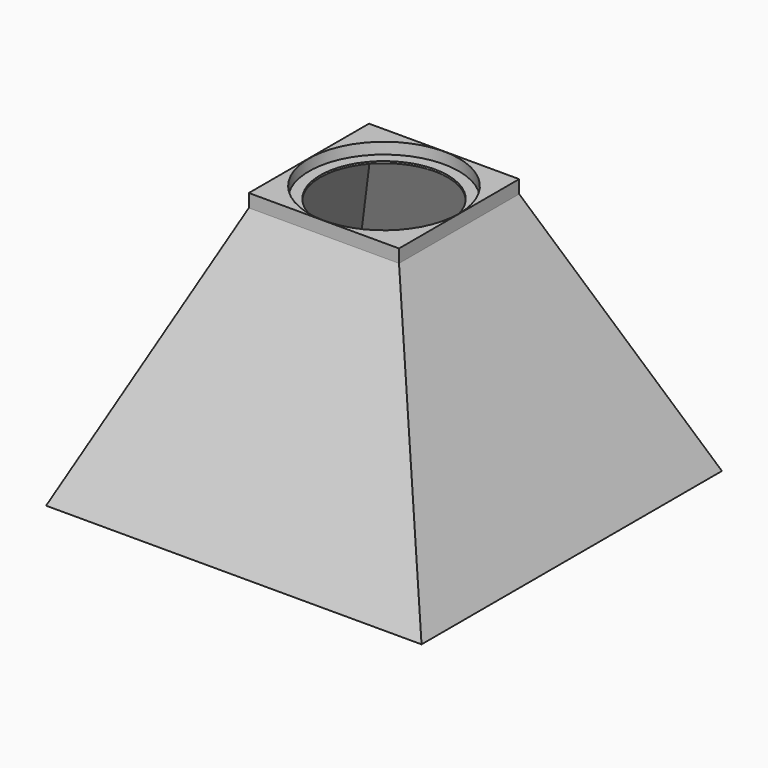
from build123d import *

# Parameters (mm, degrees)
F0_W      = 100
F0_H      = 100
F4_W      = 40
F4_H      = 40
F8_W      = 94
F8_H      = 94
F9_W      = 34
F9_H      = 34
F11_W     = 40
F11_H     = 40
F11_R     = 17
F12_DEPTH = 3.5
F13_R     = 19.95
F14_DEPTH = 3


with BuildPart() as f7:
    # F0 (on Top) → F7 section 0
    with BuildSketch(Plane.XY):
        Rectangle(F0_W, F0_H)
    # F4 (on line) → F7 section 1
    with BuildSketch(Plane(origin=(0, 0, 67.3811032171), x_dir=(1, 0, 0), z_dir=(0, 0, -1))):
        Rectangle(F4_W, F4_H)
    loft()

    # F8 (on face) → F10 section 0
    with BuildSketch(Plane(origin=(0, 0, 0), x_dir=(1, 0, 0), z_dir=(0, 0, -1))):
        Rectangle(F8_W, F8_H)
    # F9 (on face) → F10 section 1
    with BuildSketch(Plane.XY.offset(67.3811032171)):
        Rectangle(F9_W, F9_H)
    loft(mode=Mode.SUBTRACT)

    # F11 (on face) → F12 (join)
    with BuildSketch(Plane(origin=(0, 0, 67.3811032171), x_dir=(1, 0, 0), z_dir=(0, 0, -1))):
        Rectangle(F11_W, F11_H)
        Circle(F11_R, mode=Mode.SUBTRACT)
    extrude(amount=-F12_DEPTH)

    # F13 (on face) → F14 (cut)
    with BuildSketch(Plane.XY.offset(70.8811032171)):
        Circle(F13_R)
    extrude(amount=-F14_DEPTH, mode=Mode.SUBTRACT)


solid = f7.part
